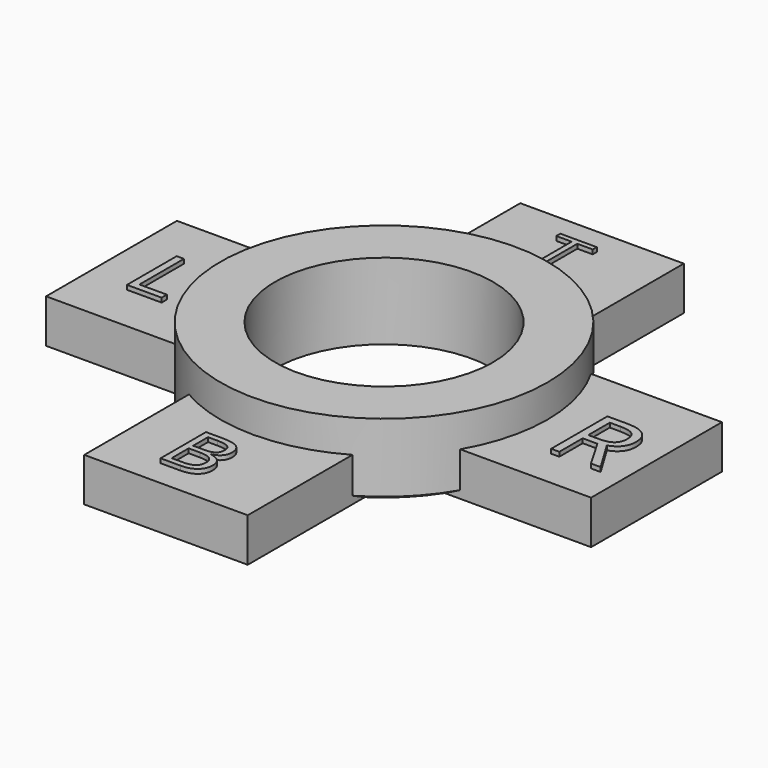
from build123d import *

# Parameters (mm, degrees)
F0_R           = 15
F0_R_2         = 10
F1_DEPTH       = 7
F3_DEPTH       = 4
F4_TEXT_SIZE   = 9.0301945521
F4_TEXT_SIZE_2 = 7.9882496114
F4_TEXT_SIZE_3 = 7.293619112
F4_TEXT_SIZE_4 = 6.2516735246
F5_DEPTH       = 0.4
F6_TEXT_SIZE   = 9.2210894864
F6_TEXT_SIZE_2 = 10.0243865745
F6_TEXT_SIZE_3 = 10.0883897782
F6_TEXT_SIZE_4 = 11.7189807093
F7_DEPTH       = 0.4
F8_T4_ANGLE    = 53.9634994863
F8_T10_ANGLE   = 53.9634994863
F8_T16_ANGLE   = 53.9634994863
F8_T22_ANGLE   = 53.9634994863


# Not quite as in the source:
# - a fillet or chamfer that OpenCascade refuses, or shapes differently, is made with other operations: its cross-section is extruded or revolved along the edge and cut away or added
# - Text() gives the source's letters only with a copy of the font that has no kerning and outlines rounded to 1/6400 em; it was checked with that copy


with BuildPart() as f1:
    # F0 (on Top) → F1 (new body)
    with BuildSketch(Plane.XY):
        Circle(F0_R)
        Circle(F0_R_2, mode=Mode.SUBTRACT)
    extrude(amount=F1_DEPTH)

    # F2 (on face) → F3 (join)
    with BuildSketch(Plane(origin=(0, 0, 0), x_dir=(1, 0, 0), z_dir=(0, 0, -1))):
        with BuildLine():
            Line((-7.5, 25), (-7.5, 12.9903810568))
            ThreePointArc((-7.5, 12.9903810568), (0, 15), (7.5, 12.9903810568))
            Line((7.5, 12.9903810568), (7.5, 25))
            Line((7.5, 25), (-7.5, 25))
        make_face()
        with BuildLine():
            Line((-25, 7.5), (-25, -7.5))
            Line((-25, -7.5), (-12.9903810568, -7.5))
            ThreePointArc((-12.9903810568, -7.5), (-15, 0), (-12.9903810568, 7.5))
            Line((-12.9903810568, 7.5), (-25, 7.5))
        make_face()
        with BuildLine():
            Line((-7.5, -25), (7.5, -25))
            Line((7.5, -25), (7.5, -12.9903810568))
            ThreePointArc((7.5, -12.9903810568), (0, -15), (-7.5, -12.9903810568))
            Line((-7.5, -12.9903810568), (-7.5, -25))
        make_face()
        with BuildLine():
            Line((25, -7.5), (25, 7.5))
            Line((25, 7.5), (12.9903810568, 7.5))
            ThreePointArc((12.9903810568, 7.5), (15, 0), (12.9903810568, -7.5))
            Line((12.9903810568, -7.5), (25, -7.5))
        make_face()
    extrude(amount=-F3_DEPTH)

    # F4 (on face) → F5 (join)
    with BuildSketch(Plane.XY.offset(4)):
        with Locations((17.620947212, -3.9669605903)):
            Text('R', F4_TEXT_SIZE, font='Open Sans', text_align=(TextAlign.LEFT, TextAlign.BOTTOM))
        with Locations((-21.8896288425, -3.0917266849)):
            Text('L', F4_TEXT_SIZE_2, font='Open Sans', text_align=(TextAlign.LEFT, TextAlign.BOTTOM))
        with Locations((-3.1346082687, -22.5969478488)):
            Text('B', F4_TEXT_SIZE_3, font='Open Sans', text_align=(TextAlign.LEFT, TextAlign.BOTTOM))
        with Locations((-1.8842730206, 18.0389285088)):
            Text('T', F4_TEXT_SIZE_4, font='Open Sans', text_align=(TextAlign.LEFT, TextAlign.BOTTOM))
    extrude(amount=F5_DEPTH)

    # F6 (on face) → F7 (cut)
    with BuildSketch(Plane(origin=(0, 0, 0), x_dir=(1, 0, 0), z_dir=(0, 0, -1))):
        with Locations(Location((2.466971986, -16.4023004472), (0, 0, 180))):
            Text('T', F6_TEXT_SIZE, font='Open Sans', text_align=(TextAlign.LEFT, TextAlign.BOTTOM))
        with Locations(Location((-16.9348176569, 4.4034924358), (0, 0, 180))):
            Text('L', F6_TEXT_SIZE_2, font='Open Sans', text_align=(TextAlign.LEFT, TextAlign.BOTTOM))
        with Locations(Location((21.6482104734, 3.9790233131), (0, 0, -180))):
            Text('R', F6_TEXT_SIZE_3, font='Open Sans', text_align=(TextAlign.LEFT, TextAlign.BOTTOM))
        with Locations(Location((3.8042876404, 22.4306331947), (0, 0, -180))):
            Text('B', F6_TEXT_SIZE_4, font='Open Sans', text_align=(TextAlign.LEFT, TextAlign.BOTTOM))
    extrude(amount=-F7_DEPTH, mode=Mode.SUBTRACT)

    # F8: chamfer of 0.7 x 1.2124355653 on 4 edges, made by hand


with BuildPart() as f8_tool2:
    # F8_s3 → F8_t4 (revolve)
    with BuildSketch(Plane(origin=(0, 0, 0), x_dir=(0, 0, 1), z_dir=(-0.9509580378, -0.3093199159, 0))):
        with BuildLine():
            Line((0.7242487113, -15.042), (-0.0242487113, -13.7455644347))
            Line((-0.0242487113, -13.7455644347), (-0.0484974226, -13.7455644347))
            ThreePointArc((-0.0484974226, -13.7455644347), (-0.0242487113, -14.3727822174), (-0.0242487113, -15))
            Line((-0.0242487113, -15), (0, -15.0242487113))
            ThreePointArc((0, -15.0242487113), (0.3621243557, -15.0242487113), (0.7242487113, -15.0662487113))
            Line((0.7242487113, -15.0662487113), (0.7242487113, -15.042))
        make_face()
    revolve(axis=Axis((0, 0, 0), (0, 0, 1)), revolution_arc=F8_T4_ANGLE)

    split(bisect_by=Plane.YZ.offset(7.5), keep=Keep.TOP)

    split(bisect_by=Plane.XZ.offset(7.5), keep=Keep.TOP)


with BuildPart() as f1_1:
    add(f1.part)

    # F8_t1: cut F8_tool2
    add(f8_tool2.part, mode=Mode.SUBTRACT)


with BuildPart() as f8_tool8:
    # F8_s9 → F8_t10 (revolve)
    with BuildSketch(Plane(origin=(0, 0, 0), x_dir=(0, 0, 1), z_dir=(0.3093199159, -0.9509580378, 0))):
        with BuildLine():
            Line((0.7242487113, -15.042), (-0.0242487113, -13.7455644347))
            Line((-0.0242487113, -13.7455644347), (-0.0484974226, -13.7455644347))
            ThreePointArc((-0.0484974226, -13.7455644347), (-0.0242487113, -14.3727822174), (-0.0242487113, -15))
            Line((-0.0242487113, -15), (0, -15.0242487113))
            ThreePointArc((0, -15.0242487113), (0.3621243557, -15.0242487113), (0.7242487113, -15.0662487113))
            Line((0.7242487113, -15.0662487113), (0.7242487113, -15.042))
        make_face()
    revolve(axis=Axis((0, 0, 0), (0, 0, 1)), revolution_arc=F8_T10_ANGLE)

    split(bisect_by=Plane.XZ.offset(-7.5), keep=Keep.BOTTOM)

    split(bisect_by=Plane.YZ.offset(7.5), keep=Keep.TOP)


with BuildPart() as f1_2:
    add(f1_1.part)

    # F8_t7: cut F8_tool8
    add(f8_tool8.part, mode=Mode.SUBTRACT)


with BuildPart() as f8_tool14:
    # F8_s15 → F8_t16 (revolve)
    with BuildSketch(Plane(origin=(0, 0, 0), x_dir=(0, 0, 1), z_dir=(0.9509580378, 0.3093199159, 0))):
        with BuildLine():
            Line((0.7242487113, -15.042), (-0.0242487113, -13.7455644347))
            Line((-0.0242487113, -13.7455644347), (-0.0484974226, -13.7455644347))
            ThreePointArc((-0.0484974226, -13.7455644347), (-0.0242487113, -14.3727822174), (-0.0242487113, -15))
            Line((-0.0242487113, -15), (0, -15.0242487113))
            ThreePointArc((0, -15.0242487113), (0.3621243557, -15.0242487113), (0.7242487113, -15.0662487113))
            Line((0.7242487113, -15.0662487113), (0.7242487113, -15.042))
        make_face()
    revolve(axis=Axis((0, 0, 0), (0, 0, 1)), revolution_arc=F8_T16_ANGLE)

    split(bisect_by=Plane.YZ.offset(-7.5), keep=Keep.BOTTOM)

    split(bisect_by=Plane.XZ.offset(-7.5), keep=Keep.BOTTOM)


with BuildPart() as f1_3:
    add(f1_2.part)

    # F8_t13: cut F8_tool14
    add(f8_tool14.part, mode=Mode.SUBTRACT)


with BuildPart() as f8_tool20:
    # F8_s21 → F8_t22 (revolve)
    with BuildSketch(Plane(origin=(0, 0, 0), x_dir=(0, 0, 1), z_dir=(-0.3093199159, 0.9509580378, 0))):
        with BuildLine():
            Line((0.7242487113, -15.042), (-0.0242487113, -13.7455644347))
            Line((-0.0242487113, -13.7455644347), (-0.0484974226, -13.7455644347))
            ThreePointArc((-0.0484974226, -13.7455644347), (-0.0242487113, -14.3727822174), (-0.0242487113, -15))
            Line((-0.0242487113, -15), (0, -15.0242487113))
            ThreePointArc((0, -15.0242487113), (0.3621243557, -15.0242487113), (0.7242487113, -15.0662487113))
            Line((0.7242487113, -15.0662487113), (0.7242487113, -15.042))
        make_face()
    revolve(axis=Axis((0, 0, 0), (0, 0, 1)), revolution_arc=F8_T22_ANGLE)

    split(bisect_by=Plane.XZ.offset(7.5), keep=Keep.TOP)

    split(bisect_by=Plane.YZ.offset(-7.5), keep=Keep.BOTTOM)


with BuildPart() as f1_4:
    add(f1_3.part)

    # F8_t19: cut F8_tool20
    add(f8_tool20.part, mode=Mode.SUBTRACT)


solid = f1_4.part
